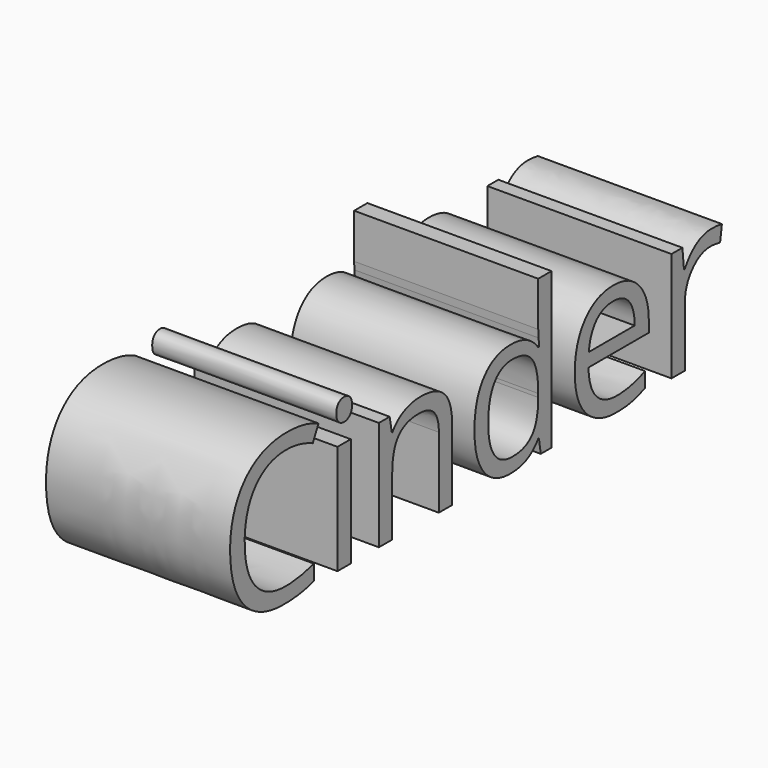
from build123d import *

# Parameters (mm, degrees)
F0_TEXT_SIZE = 14.1111111111
F1_DEPTH     = 12.7


# Not quite as in the source:
# - Text() gives the source's letters only with a copy of the font that has no kerning and outlines rounded to 1/6400 em; it was checked with that copy


with BuildPart() as f1:
    # F0 (on Right) → F1 (new body)
    with BuildSketch(Plane.YZ):
        with Locations((-27.7559408068, 13.9884060381)):
            Text('Cinder', F0_TEXT_SIZE, font='Open Sans', text_align=(TextAlign.LEFT, TextAlign.BOTTOM))
    extrude(amount=F1_DEPTH)


solid = f1.part
